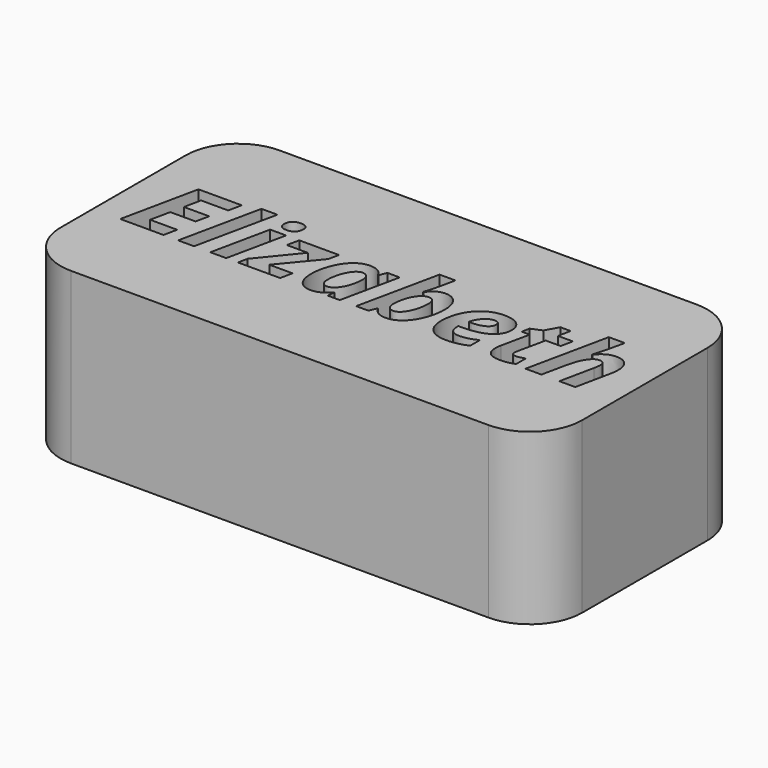
from build123d import *

# Parameters (mm, degrees)
F0_W         = 50.8
F0_H         = 25.4
F1_DEPTH     = 16.51
F2_TEXT_SIZE = 10.5546140629
F3_DEPTH     = 38.1
F4_R         = 5.08


# Not quite as in the source:
# - Text() gives the source's letters only with a copy of the font that has no kerning and outlines rounded to 1/6400 em; it was checked with that copy


with BuildPart() as f1:
    # F0 (on Top) → F1 (new body)
    with BuildSketch(Plane.XY):
        with Locations((25.4, 12.7)):
            Rectangle(F0_W, F0_H)
    extrude(amount=F1_DEPTH)

    # F2 (on face) → F3 (cut)
    with BuildSketch(Plane.XY.offset(16.51)):
        with Locations((2.3883599788, 9.0093910694)):
            Text('Elizabeth', F2_TEXT_SIZE, font='Open Sans', font_style=FontStyle.BOLDITALIC, text_align=(TextAlign.LEFT, TextAlign.BOTTOM))
    extrude(amount=-F3_DEPTH, mode=Mode.SUBTRACT)

    # F4
    f4_edges = [f1.edges().sort_by_distance(p)[0] for p in [
        (0, 0, 8.255),
        (50.8, 0, 8.255),
        (50.8, 25.4, 8.255),
        (0, 25.4, 8.255),
    ]]
    fillet(f4_edges, radius=F4_R)


solid = f1.part
